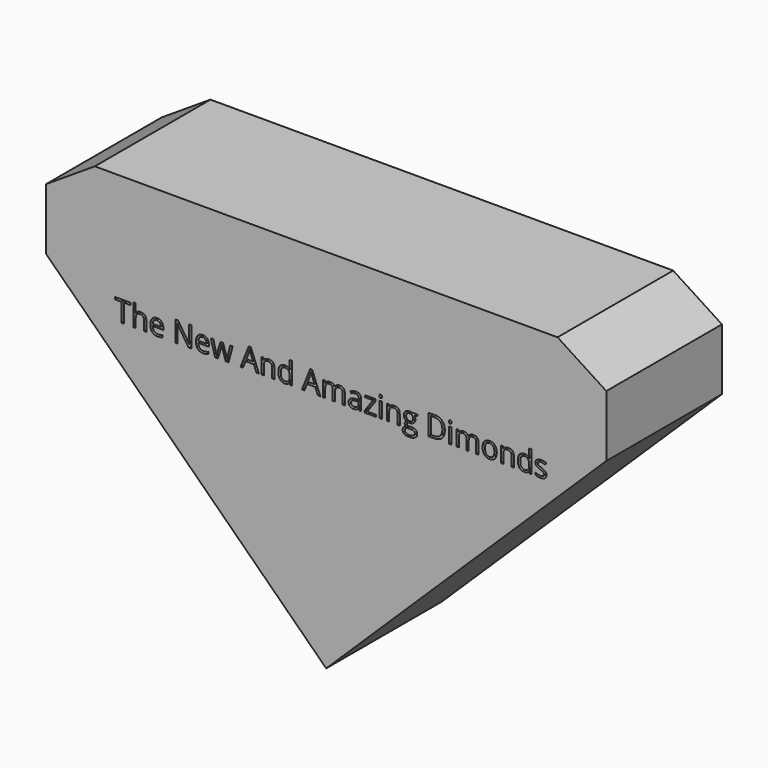
from build123d import *

# Parameters (mm, degrees)
F1_DEPTH     = 25.4
F2_TEXT_SIZE = 5.0936360883
F3_DEPTH     = 25.4


# Not quite as in the source:
# - Text() gives the source's letters only with a copy of the font that has no kerning and outlines rounded to 1/6400 em; it was checked with that copy


with BuildPart() as f1:
    # F0 (on Front) → F1 (new body)
    with BuildSketch(Plane.XZ):
        Polygon((-49.2318533361, 29.9859009683), (-49.2318533361, 19.1773027182), (0, -28.9341490716), (49.2318533361, 19.1773027182), (49.2318533361, 29.9859009683), (40.664061904, 35.5220139027), (0, 35.5220139027), (-40.664061904, 35.5220139027), align=None)
    extrude(amount=F1_DEPTH)

    # F2 (on face) → F3 (cut)
    with BuildSketch(Plane.XZ.offset(25.4)):
        with Locations((-37.1543009877, 12.831512827)):
            Text('The New And Amazing Dimonds', F2_TEXT_SIZE, font='Open Sans', text_align=(TextAlign.LEFT, TextAlign.BOTTOM))
    extrude(amount=-F3_DEPTH, mode=Mode.SUBTRACT)


solid = f1.part
